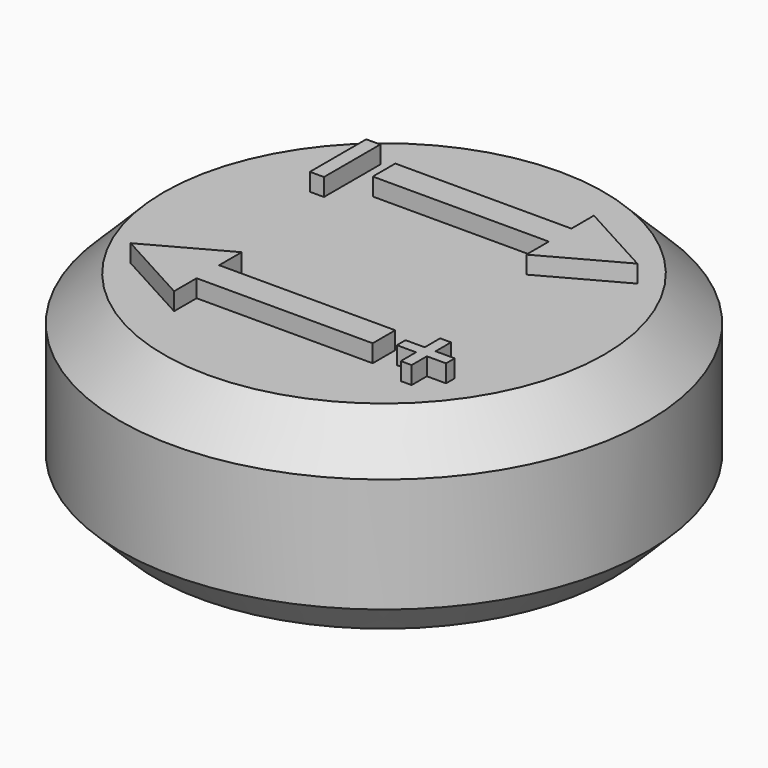
from build123d import *

# Parameters (mm, degrees)
F0_R         = 15
F1_DEPTH     = 11
F3_DEPTH     = 7
F4_SIZE      = 2.5
F5_SIZE      = 2
F6_W         = 10
F6_H         = 1.6
F6_W_2       = 0.8
F6_H_2       = 4
F6_TEXT_SIZE = 5.7636444884
F7_DEPTH     = 1


# Not quite as in the source:
# - Text() gives the source's letters only with a copy of the font that has no kerning and outlines rounded to 1/6400 em; it was checked with that copy


with BuildPart() as f1:
    # F0 (on Top) → F1 (new body)
    with BuildSketch(Plane.XY):
        Circle(F0_R)
    extrude(amount=F1_DEPTH)

    # F2 (on face) → F3 (cut)
    with BuildSketch(Plane(origin=(0, 0, 0), x_dir=(1, 0, 0), z_dir=(0, 0, -1))):
        with BuildLine():
            Line((1.2, -3.0740852298), (1.2, 3.0740852298))
            ThreePointArc((1.2, 3.0740852298), (-3.3, 0), (1.2, -3.0740852298))
        make_face()
    extrude(amount=-F3_DEPTH, mode=Mode.SUBTRACT)

    # F4
    f4_edges = [f1.edges().sort_by_distance(p)[0] for p in [
        (-15, 0, 11),
    ]]
    chamfer(f4_edges, length=F4_SIZE)

    # F5
    f5_edges = [f1.edges().sort_by_distance(p)[0] for p in [
        (-15, 0, 0),
    ]]
    chamfer(f5_edges, length=F5_SIZE)

    # F6 (on face) → F7 (join)
    with BuildSketch(Plane.XY.offset(11)):
        with Locations((0, -6.2530869618)):
            Rectangle(F6_W, F6_H)
        Polygon((-5, -7.0530869618), (-5, -5.4530869618), (-5, -3.8530869618), (-9.3863424399, -6.2530869618), (-5, -8.6530869618), align=None)
        with Locations((0, 6.2530869618)):
            Rectangle(F6_W, F6_H)
        Polygon((5, 8.6530869618), (5, 7.0530869618), (5, 5.4530869618), (5, 3.8530869618), (9.3863424399, 6.2530869618), align=None)
        with Locations((-7.0625890322, 6.066797629)):
            Rectangle(F6_W_2, F6_H_2)
        with Locations((5.7040606625, -8.2495989045)):
            Text('+', F6_TEXT_SIZE, font='Open Sans', font_style=FontStyle.BOLD, text_align=(TextAlign.LEFT, TextAlign.BOTTOM))
    extrude(amount=F7_DEPTH)


solid = f1.part
